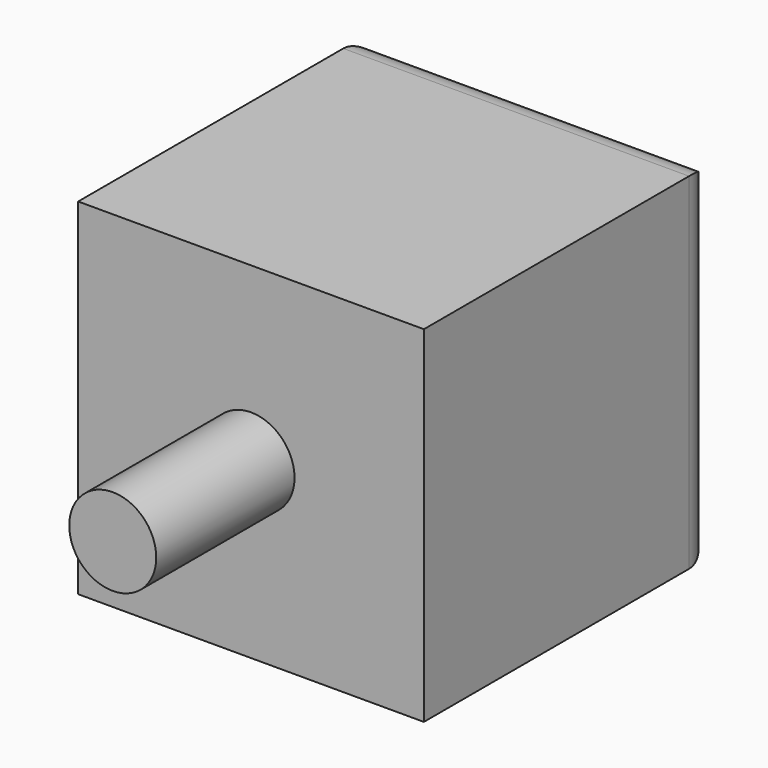
from build123d import *

# Parameters (mm, degrees)
F0_W     = 25.4
F0_H     = 25.4
F1_DEPTH = 38.1
F2_R     = 3.1962081395
F3_DEPTH = 12.7
F4_SIZE  = 12.69999
F5_R     = 2.54


# Not quite as in the source:
# - a fillet or chamfer is up to 0.001 mm smaller than in the source, because OpenCascade refuses the exact size


with BuildPart() as f1:
    # F0 (on Front) → F1 (new body)
    with BuildSketch(Plane.XZ):
        with Locations((-10.8844147762, 4.0432729903)):
            Rectangle(F0_W, F0_H)
    extrude(amount=F1_DEPTH)

    # F2 (on face) → F3 (join)
    with BuildSketch(Plane.XZ.offset(38.1)):
        with Locations((-10.8844147762, 4.0432729903)):
            Circle(F2_R)
    extrude(amount=F3_DEPTH)

    # F4 (size 12.7 in the source; OpenCascade refuses exactly that, so slightly less here)
    f4_edges = [f1.edges().sort_by_distance(p)[0] for p in [
        (-10.884415, 0, 16.743273),
        (-10.884415, 0, -8.656727),
        (1.815585, 0, 4.043273),
        (-23.584415, 0, 4.043273),
    ]]
    chamfer(f4_edges, length=F4_SIZE)

    # F5
    f5_edges = [f1.edges().sort_by_distance(p)[0] for p in [
        (-23.584415, -12.69999, 4.043273),
        (-10.884415, -12.69999, 16.743273),
        (1.815585, -12.69999, 4.043273),
        (-10.884415, -12.69999, -8.656727),
    ]]
    fillet(f5_edges, radius=F5_R)


solid = f1.part
